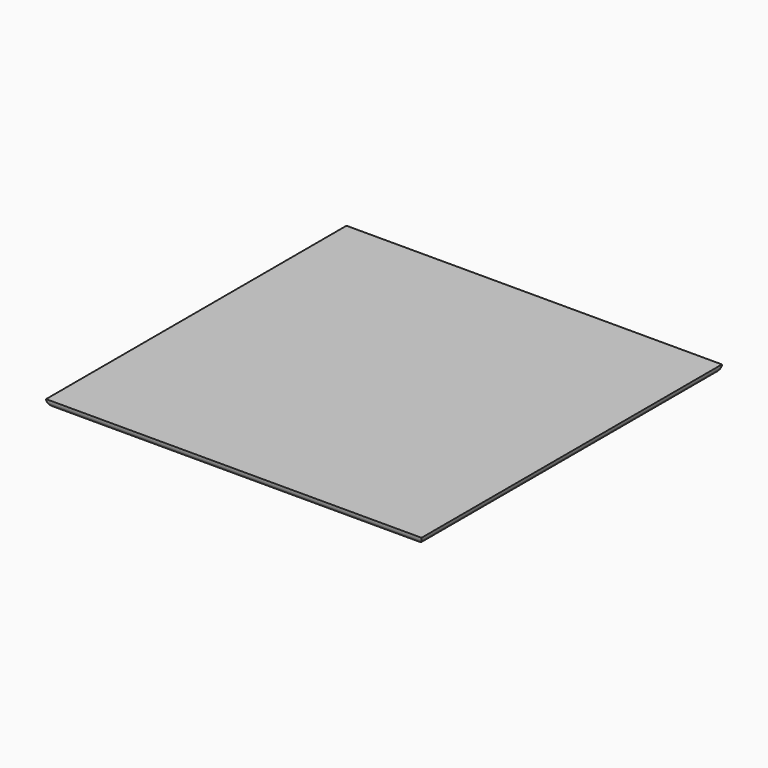
from build123d import *

# Parameters (mm, degrees)
F0_W     = 144
F0_H     = 144
F1_DEPTH = 3
F2_R     = 2.99999


# Not quite as in the source:
# - a fillet or chamfer is up to 0.001 mm smaller than in the source, because OpenCascade refuses the exact size


with BuildPart() as f1:
    # F0 (on Top) → F1 (new body)
    with BuildSketch(Plane.XY):
        with Locations((72, -72)):
            Rectangle(F0_W, F0_H)
    extrude(amount=F1_DEPTH)

    # F2 (radius 3 in the source; OpenCascade refuses exactly that, so slightly less here)
    f2_edges = [f1.edges().sort_by_distance(p)[0] for p in [
        (72, 0, 0),
        (0, -72, 0),
        (72, -144, 0),
        (144, -72, 0),
    ]]
    fillet(f2_edges, radius=F2_R)


solid = f1.part
